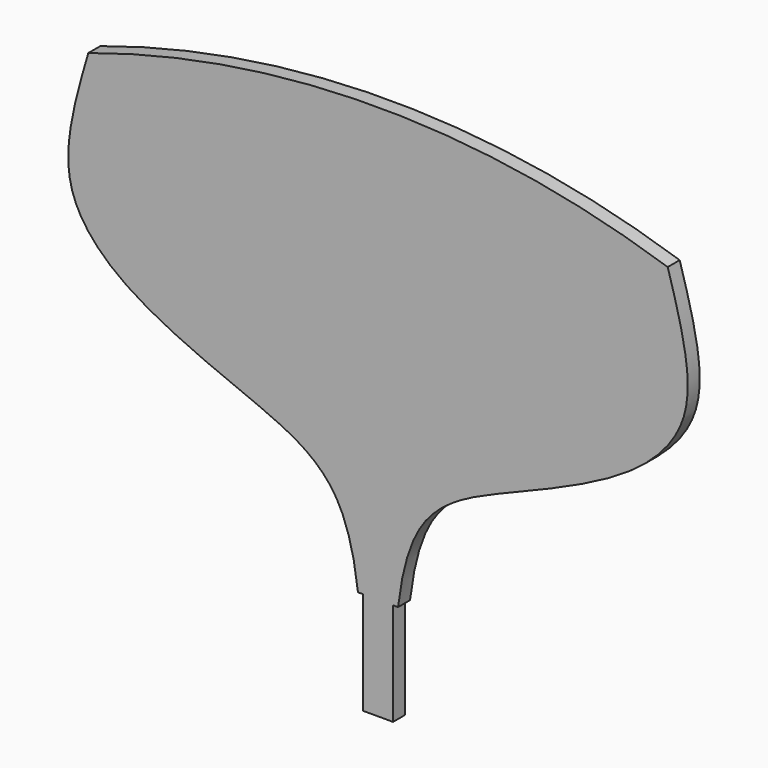
from build123d import *

# Parameters (mm, degrees)
F0_W     = 38.2413167982
F0_H     = 130.5519748793
F1_DEPTH = 19.05


with BuildPart() as f1:
    # F0 (on Front) → F1 (new body)
    with BuildSketch(Plane.XZ):
        with Locations((-5e-10, 64.9347287138)):
            Rectangle(F0_W, F0_H)
        with BuildLine():
            Line((-19.1206583996, 130.2107161535), (19.1206583986, 130.2107161535))
            Line((19.1206583986, 130.2107161535), (25.4706583986, 130.2107161535))
            add(Edge.make_bspline(
                [(25.4706583986, 130.2107161535), (30.0724719756, 169.0966659039), (51.3980125218, 257.0949252577), (168.2834825455, 304.8190286771), (326.925094009, 369.4938490194), (396.8974330576, 452.268946401), (393.7810574923, 535.008276766), (377.0494931199, 592.3264271799), (368.2999999833, 622.3000000618)],
                knots=[0.1131891299, 0.1131891299, 0.1131891299, 0.1131891299, 0.2225944071, 0.3940346608, 0.5865569639, 0.732236582, 0.8599775765, 1, 1, 1, 1], degree=3))
            ThreePointArc((368.2999999833, 622.3000000618), (-1.67e-08, 681.4277668685), (-368.3000000167, 622.3000000618))
            add(Edge.make_bspline(
                [(-25.4706584275, 130.2107161535), (-30.0724720137, 169.0966658909), (-51.3980125817, 257.094925206), (-168.2834825322, 304.8190286898), (-326.9250939954, 369.4938490451), (-396.8974330089, 452.2689464188), (-393.781057464, 535.008276759), (-377.0494931536, 592.3264271786), (-368.3000000167, 622.3000000618)],
                knots=[0.1131891299, 0.1131891299, 0.1131891299, 0.1131891299, 0.222594407, 0.3940346608, 0.5865569639, 0.7322365819, 0.8599775765, 1, 1, 1, 1], degree=3))
            Line((-25.4706584275, 130.2107161535), (-19.1206583996, 130.2107161535))
        make_face()
    extrude(amount=F1_DEPTH)


solid = f1.part
